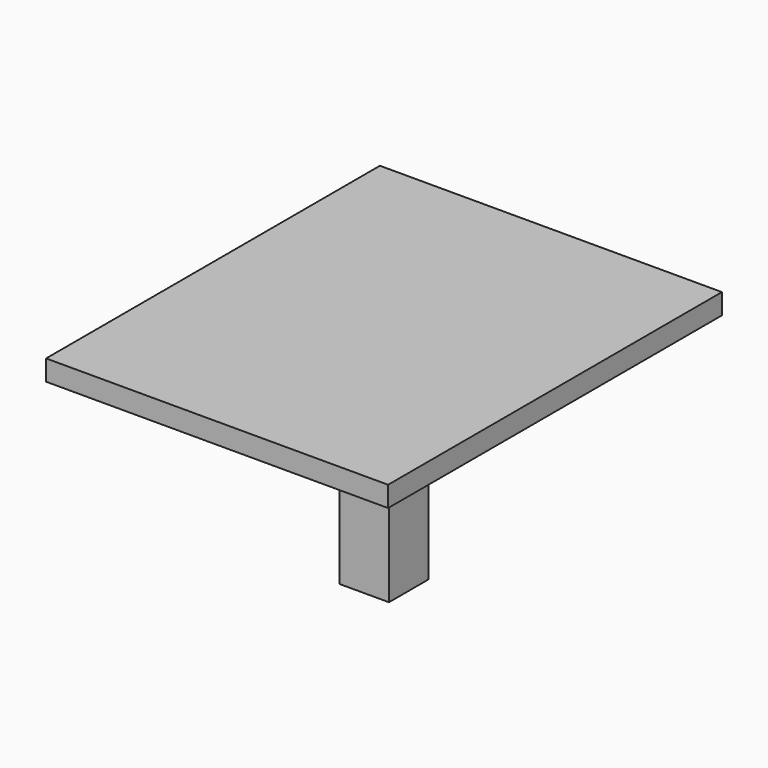
from build123d import *

# Parameters (mm, degrees)
F0_W          = 184.15
F0_H          = 184.15
F1_DEPTH      = 762
F5_R          = 12.7
F5_R_2        = 9.525
F6_DEPTH      = 355.6
F6_DEPTH_BACK = 88.9
F7_COUNT      = 4
F8_W          = 1270
F8_H          = 1549.4
F9_DEPTH      = 76.2


with BuildPart() as f1:
    # F0 (on Top) → F1 (new body)
    with BuildSketch(Plane.XY):
        Rectangle(F0_W, F0_H)
    extrude(amount=F1_DEPTH)

    # F5 (on line) → F6 (join, two sides)
    with BuildSketch(Plane(origin=(0, -353.9190367264, 353.9190367264), x_dir=(1, 0, 0), z_dir=(0, -0.7071067812, 0.7071067812))) as f6_sk:
        with Locations((0, 294.103387965)):
            Circle(F5_R)
        with Locations((0, 294.103387965)):
            Circle(F5_R_2, mode=Mode.SUBTRACT)
    extrude(amount=F6_DEPTH)
    extrude(f6_sk.sketch, amount=-F6_DEPTH_BACK)


with BuildPart() as f7_1:
    # F7: instance of F1
    add(f1.part.rotate(Axis((0, 0, 576.6244882105), (0, 0, -1)), 1 * 360 / F7_COUNT))


with BuildPart() as f7_2:
    # F7: instance of F1
    add(f1.part.rotate(Axis((0, 0, 576.6244882105), (0, 0, -1)), 2 * 360 / F7_COUNT))


with BuildPart() as f7_3:
    # F7: instance of F1
    add(f1.part.rotate(Axis((0, 0, 576.6244882105), (0, 0, -1)), 3 * 360 / F7_COUNT))


with BuildPart() as f1_1:
    add(f1.part)

    # F8 (on face) → F9 (join)
    with BuildSketch(Plane.XY.offset(762)):
        Rectangle(F8_W, F8_H)
    extrude(amount=F9_DEPTH)


solid = Compound([f7_1.part, f7_2.part, f7_3.part, f1_1.part])
